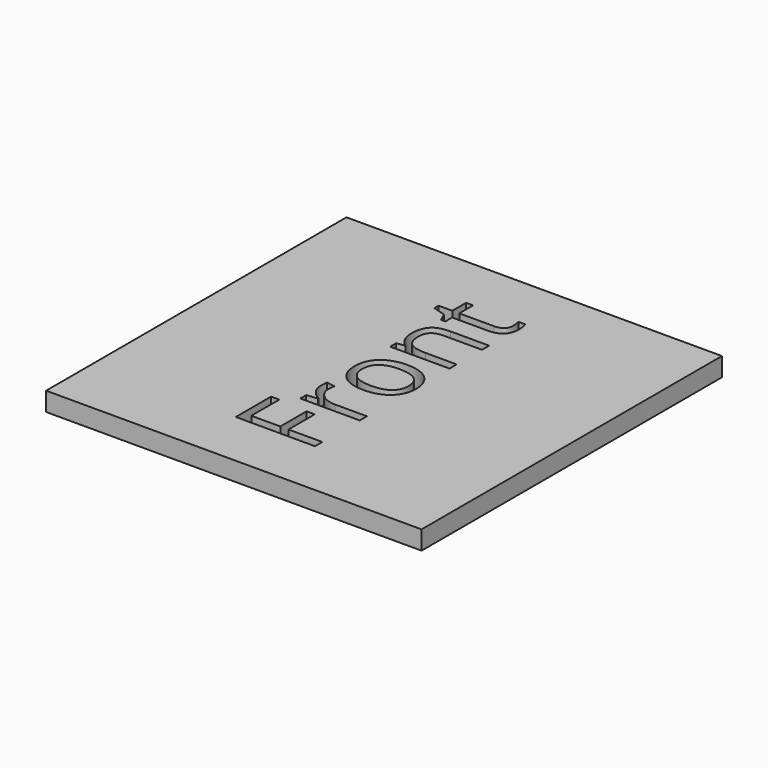
from build123d import *

# Parameters (mm, degrees)
F0_W         = 100
F0_H         = 100
F1_DEPTH     = 5
F2_TEXT_SIZE = 29.5384615385
F3_DEPTH     = 5


# Not quite as in the source:
# - Text() gives the source's letters only with a copy of the font that has no kerning and outlines rounded to 1/6400 em; it was checked with that copy


with BuildPart() as f1:
    # F0 (on Top) → F1 (new body)
    with BuildSketch(Plane.XY):
        Rectangle(F0_W, F0_H)
    extrude(amount=F1_DEPTH)

    # F2 (on face) → F3 (cut)
    with BuildSketch(Plane.XY.offset(5)):
        with Locations(Location((9.2933333356, -37.5), (0, 0, 90))):
            Text('Front', F2_TEXT_SIZE, font='Open Sans', text_align=(TextAlign.LEFT, TextAlign.BOTTOM))
    extrude(amount=-F3_DEPTH, mode=Mode.SUBTRACT)


solid = f1.part
